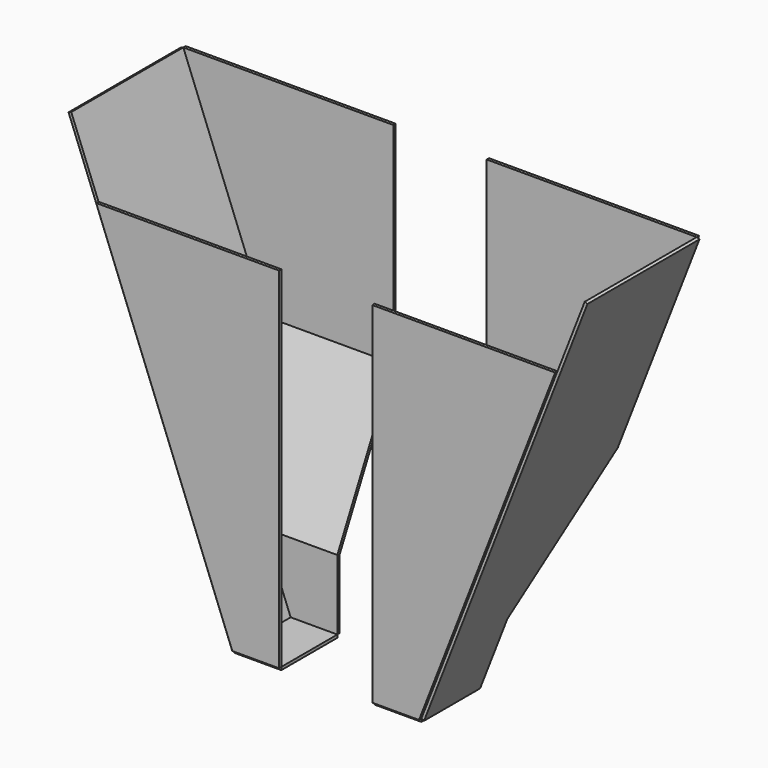
from build123d import *

# Parameters (mm, degrees)
F6_DEPTH  = 2.54
F8_DEPTH  = 3.175
F9_DEPTH  = 3.175
F10_DEPTH = 3.175
F11_DEPTH = 3.175
F13_DEPTH = 3.175
F15_W     = 50.8
F15_H     = 76.2
F16_DEPTH = 3.175


# Not quite as in the source:
# - ends of sketch curves that miss each other by under 0.0002 mm in the source are joined


with BuildPart() as f6:
    # F5 (on Right) → F6 (new body)
    with BuildSketch(Plane.YZ):
        Polygon((-76.2, 76.2), (0, 76.2), (0, 228.6), align=None)
    extrude(amount=-F6_DEPTH)


with BuildPart() as f8:
    # F1 (on offset) → F8 (new body)
    with BuildSketch(Plane.XZ.offset(152.4)):
        Polygon((0, 381), (0, 0), (50.8, 0), (198.9666666121, 381), align=None)
    extrude(amount=F8_DEPTH)


with BuildPart() as f9:
    # F4 (on Front) → F9 (new body)
    with BuildSketch(Plane.XZ):
        Polygon((228.6, 457.2), (0, 457.2), (0, 228.6), (139.7000000328, 228.6), align=None)
    extrude(amount=-F9_DEPTH)


with BuildPart() as f10:
    # F3 (on offset) → F10 (new body)
    with BuildSketch(Plane.XZ.offset(76.2)):
        Polygon((0, 76.2), (0, 0), (50.8, 0), (80.4333333224, 76.2), align=None)
    extrude(amount=-F10_DEPTH)


with BuildPart() as f11:
    # F7 (on face) → F11 (new body)
    with BuildSketch(Plane(origin=(0, -91.44, 45.72), x_dir=(1, 0, 0), z_dir=(0, -0.894427191, 0.4472135955))):
        Polygon((0, 204.4660558626), (0, 34.0776759771), (80.4333418, 34.0776759771), (139.7, 204.4660558626), align=None)
    extrude(amount=-F11_DEPTH)


with BuildPart() as f13:
    # F12 (on face) → F13 (new body)
    with BuildSketch(Plane(origin=(44.1265415592, 0, -17.1603217112), x_dir=(0, 1, 0), z_dir=(0.9320046716, 0, -0.362446261))):
        Polygon((-152.4, 427.2085042593), (-152.4, 18.4122700608), (-76.2, 18.4122700608), (-76.2, 100.1715169005), (0, 263.6900105918), (0, 508.9677511228), (-152.4, 508.9677511228), align=None)
    extrude(amount=F13_DEPTH)


with BuildPart() as f16:
    # F15 (on face) → F16 (new body)
    with BuildSketch(Plane(origin=(0, 0, 0), x_dir=(1, 0, 0), z_dir=(0, 0, -1))):
        with Locations((25.4, 114.3)):
            Rectangle(F15_W, F15_H)
    extrude(amount=F16_DEPTH)


with BuildPart() as f17_1:
    # F17: instance of F9
    add(f9.part.mirror(Plane.YZ.offset(-50.8)))


with BuildPart() as f17_2:
    # F17: instance of F13
    add(f13.part.mirror(Plane.YZ.offset(-50.8)))


with BuildPart() as f17_3:
    # F17: instance of F8
    add(f8.part.mirror(Plane.YZ.offset(-50.8)))


with BuildPart() as f17_4:
    # F17: instance of F10
    add(f10.part.mirror(Plane.YZ.offset(-50.8)))


with BuildPart() as f17_5:
    # F17: instance of F16
    add(f16.part.mirror(Plane.YZ.offset(-50.8)))


with BuildPart() as f17_6:
    # F17: instance of F11
    add(f11.part.mirror(Plane.YZ.offset(-50.8)))


solid = Compound([f6.part, f8.part, f9.part, f10.part, f11.part, f13.part, f16.part, f17_1.part, f17_2.part, f17_3.part, f17_4.part, f17_5.part, f17_6.part])
